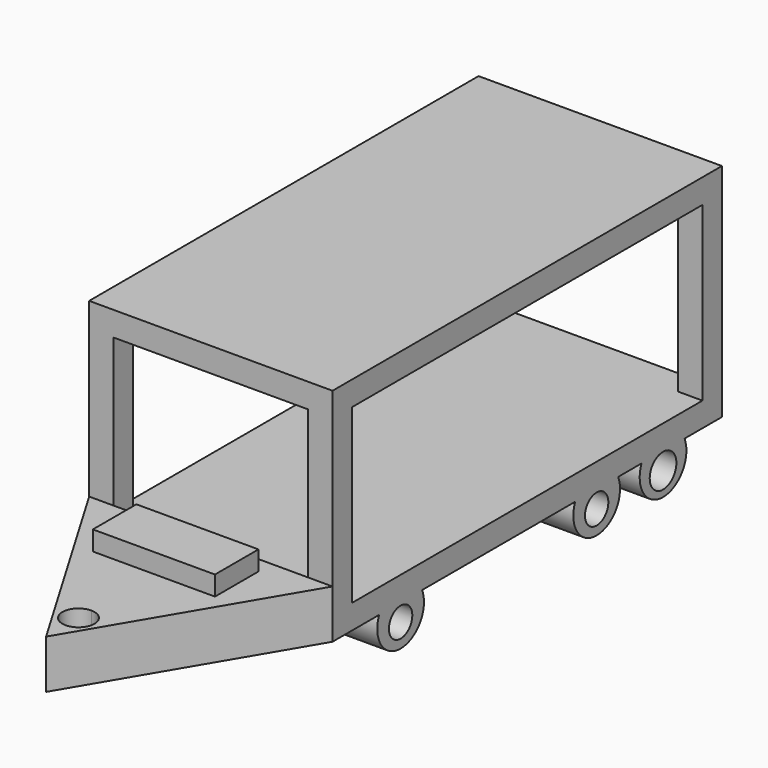
from build123d import *

# Parameters (mm, degrees)
F0_W      = 63.5
F0_H      = 127
F1_DEPTH  = 57.658
F2_W      = 50.7999993861
F2_H      = 114.3
F3_DEPTH  = 155.702
F4_W      = 114.3000005424
F4_H      = 44.9580000767
F5_DEPTH  = 96.774
F6_W      = 50.8000007063
F6_H      = 44.9580000767
F7_DEPTH  = 127
F8_DEPTH  = 120.142
F9_DEPTH  = 115.824
F11_DEPTH = 12.7
F13_DEPTH = 25.4
F14_W     = 31.8544553593
F14_H     = 14.1892433167
F15_DEPTH = 5.08
F16_R     = 4.3491356376
F16_R_2   = 3.81
F17_DEPTH = 63.5
F18_DEPTH = 94.488


# Not quite as in the source:
# - after a boolean that leaves OpenCascade's solid faulty, fix() repairs it


with BuildPart() as f1:
    # F0 (on Top) → F1 (new body)
    with BuildSketch(Plane.XY):
        with Locations((4.1889519542, 37.7824994028)):
            Rectangle(F0_W, F0_H)
    extrude(amount=F1_DEPTH)

    # F2 (on face) → F3 (cut)
    with BuildSketch(Plane.XY.offset(57.658)):
        with Locations((4.1889529675, 37.7824994028)):
            Rectangle(F2_W, F2_H)
    extrude(amount=-F3_DEPTH, mode=Mode.SUBTRACT)

    # F4 (on face) → F5 (cut)
    with BuildSketch(Plane.YZ.offset(35.9389519542)):
        with Locations((37.7824991316, 28.8289999616)):
            Rectangle(F4_W, F4_H)
    extrude(amount=-F5_DEPTH, mode=Mode.SUBTRACT)

    # F6 (on face) → F7 (cut)
    with BuildSketch(Plane(origin=(0, 101.2824994028, 0), x_dir=(-1, 0, 0), z_dir=(0, 1, 0))):
        with Locations((-4.1889523074, 28.8289999616)):
            Rectangle(F6_W, F6_H)
    extrude(amount=-F7_DEPTH, mode=Mode.SUBTRACT)

    add(f1.part.fix(), mode=Mode.REPLACE)

    # F8 (add): a face of the model
    f8_faces = [f1.faces().sort_by_distance(p)[0] for p in [
        (4.1889529675, -19.3675005972, 3.1749999616),
    ]]
    extrude(f8_faces, amount=F8_DEPTH)

    # F9 (add): a face of the model
    f9_faces = [f1.faces().sort_by_distance(p)[0] for p in [
        (4.1889529675, -19.3675005972, 54.483),
    ]]
    extrude(f9_faces, amount=F9_DEPTH)

    # F10 (on Top) → F11 (join)
    with BuildSketch(Plane.XY):
        Polygon((4.1889519542, -25.7175005972), (-27.5610480458, -25.7175005972), (4.1889519542, -79.4553607702), align=None)
        Polygon((35.9389519542, -25.7175005972), (4.1889519542, -25.7175005972), (4.1889519542, -79.4553607702), align=None)
    extrude(amount=F11_DEPTH)

    # F12 (on face) → F13 (cut)
    with BuildSketch(Plane.XY.offset(12.7)):
        with BuildLine():
            Line((4.1889519963, -73.0581155537), (4.1889520512, -64.701584864))
            ThreePointArc((4.1889520512, -64.701584864), (-0.0063655555, -68.8798501813), (4.1889519963, -73.0581155537))
        make_face()
        with BuildLine():
            ThreePointArc((4.1889519963, -73.0581155537), (7.1324492077, -71.8283317208), (8.3502344445, -68.8798502088))
            ThreePointArc((8.3502344445, -68.8798502088), (7.1324492271, -65.9313687162), (4.1889520512, -64.701584864))
            Line((4.1889520512, -64.701584864), (4.1889519963, -73.0581155537))
        make_face()
    extrude(amount=-F13_DEPTH, mode=Mode.SUBTRACT)

    # F14 (on face) → F15 (join)
    with BuildSketch(Plane.XY.offset(12.7)):
        with Locations((4.1026878171, -37.0831862092)):
            Rectangle(F14_W, F14_H)
    extrude(amount=F15_DEPTH)

    # F16 (on face) → F17 (join)
    with BuildSketch(Plane(origin=(-27.5610480458, 0, 0), x_dir=(0, -1, 0), z_dir=(-1, 0, 0))):
        with BuildLine():
            Line((-75.0678375838, 0), (-89.0953838825, 0))
            ThreePointArc((-89.0953838825, 0), (-82.0816107331, -10.598487235), (-75.0678375838, 0))
        make_face()
        with Locations((-82.0816107331, -4.520711489)):
            Circle(F16_R, mode=Mode.SUBTRACT)
        with BuildLine():
            Line((-53.4179941057, 0), (-67.4455404045, 0))
            ThreePointArc((-67.4455404045, 0), (-60.4317672551, -10.598487235), (-53.4179941057, 0))
        make_face()
        with Locations((-60.4317672551, -4.520711489)):
            Circle(F16_R_2, mode=Mode.SUBTRACT)
        with BuildLine():
            Line((10.5258625229, 0), (-3.5016837758, 0))
            ThreePointArc((-3.5016837758, 0), (3.5120893735, -10.598487235), (10.5258625229, 0))
        make_face()
        with Locations((3.5120893735, -4.520711489)):
            Circle(F16_R_2, mode=Mode.SUBTRACT)
        with Locations((-82.0816107331, -4.520711489)):
            Circle(F16_R)
        with Locations((-60.4317672551, -4.520711489)):
            Circle(F16_R_2)
        with Locations((3.5120893735, -4.520711489)):
            Circle(F16_R_2)
    extrude(amount=-F17_DEPTH)

    # F16 (on face) → F18 (cut)
    with BuildSketch(Plane(origin=(-27.5610480458, 0, 0), x_dir=(0, -1, 0), z_dir=(-1, 0, 0))):
        with Locations((-82.0816107331, -4.520711489)):
            Circle(F16_R)
        with Locations((-60.4317672551, -4.520711489)):
            Circle(F16_R_2)
        with Locations((3.5120893735, -4.520711489)):
            Circle(F16_R_2)
    extrude(amount=-F18_DEPTH, mode=Mode.SUBTRACT)


solid = f1.part
